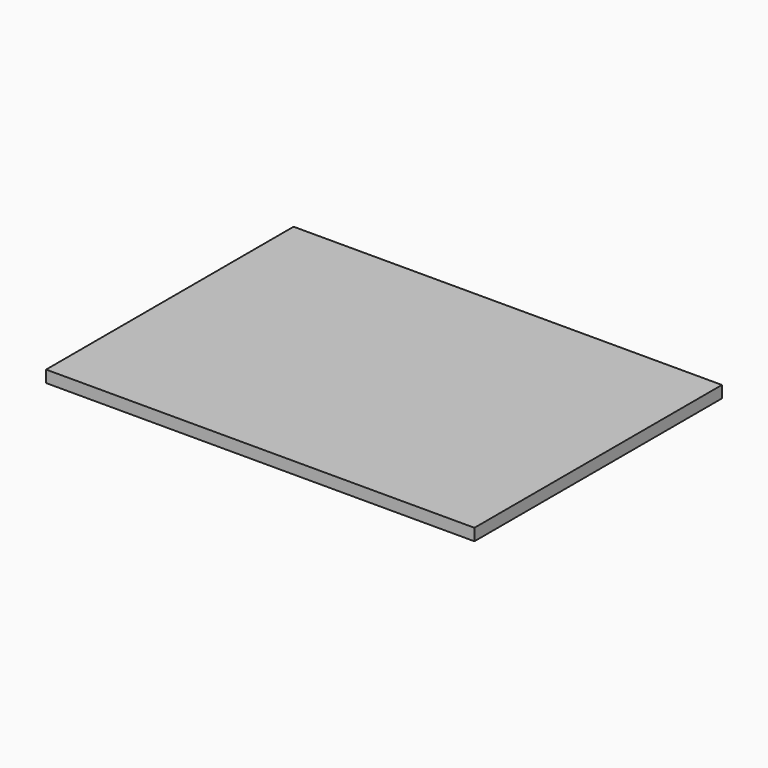
from build123d import *

# Parameters (mm, degrees)
F0_W     = 1040
F0_H     = 40
F1_DEPTH = 1440


# Not quite as in the source:
# - a feature of the source that left no trace in its solid (it failed there, or was rolled back) is left out


with BuildPart() as f1:
    # F0 (on Right) → F1 (new body)
    with BuildSketch(Plane.YZ):
        with Locations((-520, 20)):
            Rectangle(F0_W, F0_H)
    extrude(amount=F1_DEPTH)


solid = f1.part
